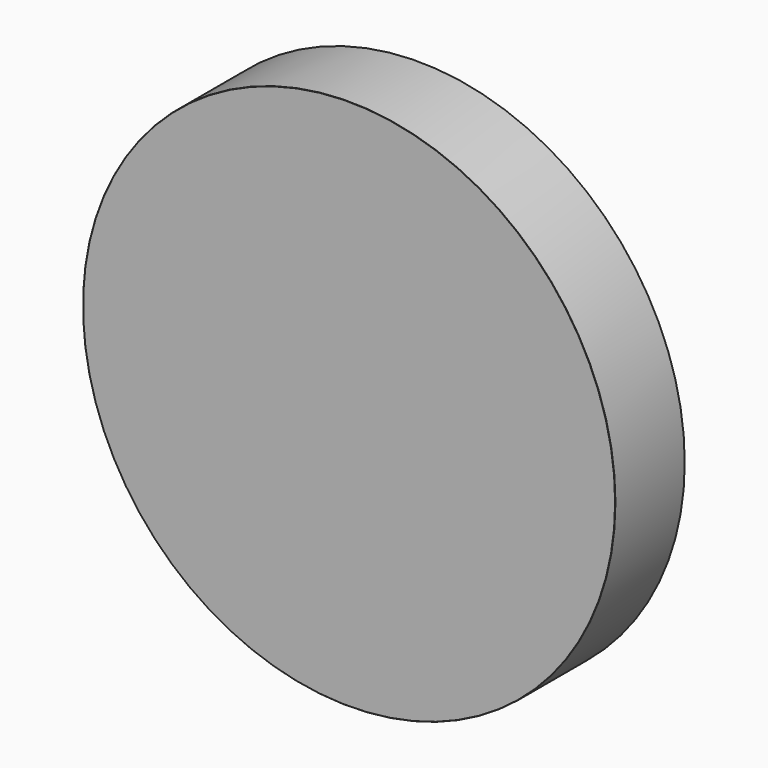
from build123d import *

# Parameters (mm, degrees)
F0_R     = 150
F1_DEPTH = 49
F2_R     = 109.5
F2_R_2   = 85.5
F2_R_3   = 31.5
F3_DEPTH = 11
F4_SIZE  = 0.1


# Not quite as in the source:
# - a feature names something its author has since deleted; it is built from what else it names


with BuildPart() as f1:
    # F0 (on Front) → F1 (new body)
    with BuildSketch(Plane.XZ):
        Circle(F0_R)
    extrude(amount=F1_DEPTH)

    # F2 (on Front) → F3 (cut)
    with BuildSketch(Plane.XZ):
        Circle(F2_R)
        Circle(F2_R_2, mode=Mode.SUBTRACT)
        Circle(F2_R_3)
    extrude(amount=F3_DEPTH, mode=Mode.SUBTRACT)

    # F4
    f4_edges = [f1.edges().sort_by_distance(p)[0] for p in [
        (-150, 0, 0),
        (150, -24.5, 0),
        (-150, -49, 0),
        (-109.5, 0, 0),
        (109.5, -5.5, 0),
        (-109.5, -11, 0),
        (-85.5, -11, 0),
        (-85.5, 0, 0),
        (85.5, -5.5, 0),
        (31.5, -5.5, 0),
        (-31.5, 0, 0),
        (-31.5, -11, 0),
    ]]
    chamfer(f4_edges, length=F4_SIZE)


solid = f1.part
